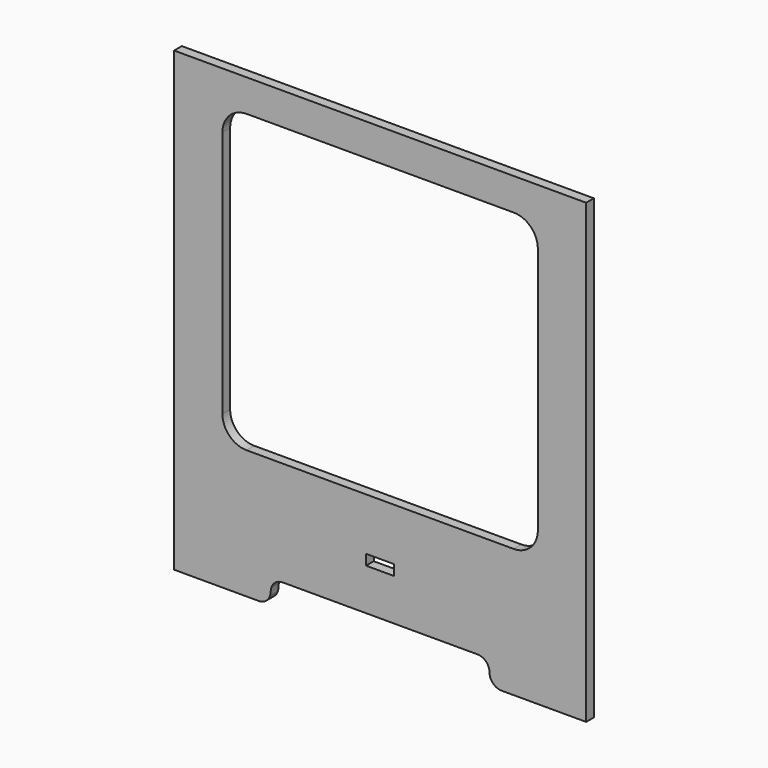
from build123d import *

# Parameters (mm, degrees)
F2_DEPTH = 12
F3_W     = 392
F3_H     = 368
F3_W_2   = 35
F3_H_2   = 13
F4_DEPTH = 12
F5_R     = 30
F6_R     = 14.99999


# Not quite as in the source:
# - a fillet or chamfer is up to 0.001 mm smaller than in the source, because OpenCascade refuses the exact size
# - a feature names something its author has since deleted; it is built from what else it names


with BuildPart() as f2:
    # F1 (on Front) → F2 (new body)
    with BuildSketch(Plane.XZ):
        Polygon((256, -284), (256, 284), (-256, 284), (-256, -284), (-136, -284), (-136, -254), (136, -254), (136, -284), align=None)
    extrude(amount=F2_DEPTH)

    # F3 (on face) → F4 (cut, through all)
    with BuildSketch(Plane.XZ.offset(12)):
        with Locations((0, 60)):
            Rectangle(F3_W, F3_H)
        with Locations((0, -195.5)):
            Rectangle(F3_W_2, F3_H_2)
    extrude(amount=-F4_DEPTH, mode=Mode.SUBTRACT)

    # F5
    f5_edges = [f2.edges().sort_by_distance(p)[0] for p in [
        (-196, -6, -124),
        (-196, -6, 244),
        (196, -6, 244),
        (196, -6, -124),
    ]]
    fillet(f5_edges, radius=F5_R)

    # F6 (radius 15 in the source; OpenCascade refuses exactly that, so slightly less here)
    f6_edges = [f2.edges().sort_by_distance(p)[0] for p in [
        (-136, -6, -284),
        (-136, -6, -254),
        (136, -6, -284),
        (136, -6, -254),
    ]]
    fillet(f6_edges, radius=F6_R)


solid = f2.part
